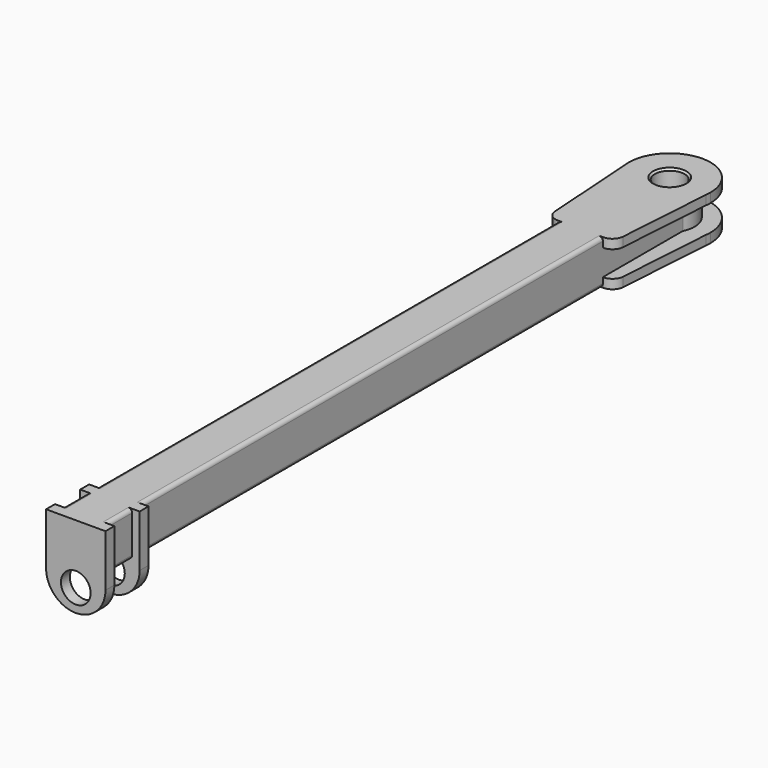
from build123d import *

# Parameters (mm, degrees)
F0_W      = 120
F0_H      = 120
F0_W_2    = 100
F0_H_2    = 100
F1_DEPTH  = 1000
F2_R      = 67.5
F3_DEPTH  = 120
F4_R      = 40
F5_DEPTH  = 120
F7_DEPTH  = 25
F9_DEPTH  = 25
F10_R     = 40
F11_DEPTH = 160
F12_W     = 30
F12_H     = 220
F13_DEPTH = 140
F14_W     = 30
F14_H     = 220
F15_DEPTH = 20
F16_W     = 30
F16_H     = 220
F17_DEPTH = 140
F18_W     = 30
F18_H     = 220
F19_DEPTH = 20
F20_R     = 40
F21_DEPTH = 145
F22_R     = 10
F23_R     = 79.99999
F24_R     = 30
F25_SIZE  = 5


# Not quite as in the source:
# - a fillet or chamfer is up to 0.001 mm smaller than in the source, because OpenCascade refuses the exact size


with BuildPart() as f1:
    # F0 (on Front) → F1 (new body, symmetric)
    with BuildSketch(Plane.XZ):
        Rectangle(F0_W, F0_H)
        Rectangle(F0_W_2, F0_H_2, mode=Mode.SUBTRACT)
    extrude(amount=F1_DEPTH, both=True)

    # F2 (on face) → F3 (join)
    with BuildSketch(Plane.XY.offset(60)):
        with Locations((0, 1000)):
            Circle(F2_R)
    extrude(amount=-F3_DEPTH)

    # F4 (on face) → F5 (cut)
    with BuildSketch(Plane.XY.offset(60)):
        with Locations((0, 1000)):
            Circle(F4_R)
    extrude(amount=-F5_DEPTH, mode=Mode.SUBTRACT)

    # F6 (on face) → F7 (join)
    with BuildSketch(Plane.XY.offset(60)):
        with BuildLine():
            Line((109.0265486726, 985.3982300885), (110, 1000))
            ThreePointArc((110, 1000), (0, 1110), (-110, 1000))
            Line((-110, 1000), (-109.0265486726, 985.3982300885))
            ThreePointArc((-109.0265486726, 985.3982300885), (0, 890), (109.0265486726, 985.3982300885))
        make_face()
        with BuildLine():
            ThreePointArc((109.0265486726, 985.3982300885), (109.7563673642, 992.6829088424), (110, 1000))
            Line((110, 1000), (109.0265486726, 985.3982300885))
        make_face()
        with BuildLine():
            Line((-109.0265486726, 985.3982300885), (-110, 1000))
            ThreePointArc((-110, 1000), (-109.7563673642, 992.6829088424), (-109.0265486726, 985.3982300885))
        make_face()
        with BuildLine():
            Line((90, 700), (109.0265486726, 985.3982300885))
            ThreePointArc((109.0265486726, 985.3982300885), (0, 890), (-109.0265486726, 985.3982300885))
            Line((-109.0265486726, 985.3982300885), (-90, 700))
            Line((-90, 700), (90, 700))
        make_face()
    extrude(amount=-F7_DEPTH)

    # F8 (on face) → F9 (join)
    with BuildSketch(Plane(origin=(0, 0, -60), x_dir=(1, 0, 0), z_dir=(0, 0, -1))):
        with BuildLine():
            Line((109.0265486726, -985.3982300885), (110, -1000))
            ThreePointArc((110, -1000), (109.7563673642, -992.6829088424), (109.0265486726, -985.3982300885))
        make_face()
        with BuildLine():
            ThreePointArc((-109.7502513746, -992.5917395282), (-3.706234531, -1109.9375451136), (110, -1000))
            Line((110, -1000), (109.0265486726, -985.3982300885))
            ThreePointArc((109.0265486726, -985.3982300885), (-3.6149109138, -890.0594141407), (-109.7502513746, -992.5917395282))
        make_face()
        with BuildLine():
            ThreePointArc((-109.7502513746, -992.5917395282), (-3.6149109138, -890.0594141407), (109.0265486726, -985.3982300885))
            Line((109.0265486726, -985.3982300885), (90, -700))
            Line((90, -700), (-90, -700))
            Line((-90, -700), (-109.7502513746, -992.5917395282))
        make_face()
    extrude(amount=-F9_DEPTH)

    # F10 (on face) → F11 (cut)
    with BuildSketch(Plane(origin=(0, 0, -60), x_dir=(1, 0, 0), z_dir=(0, 0, -1))):
        with Locations((0, -1000)):
            Circle(F10_R)
    extrude(amount=-F11_DEPTH, mode=Mode.SUBTRACT)

    # F12 (on face) → F13 (join)
    with BuildSketch(Plane.YZ.offset(60)):
        with Locations((-870, -50)):
            Rectangle(F12_W, F12_H)
    extrude(amount=-F13_DEPTH)

    # F14 (on face) → F15 (join)
    with BuildSketch(Plane.YZ.offset(60)):
        with Locations((-870, -50)):
            Rectangle(F14_W, F14_H)
    extrude(amount=F15_DEPTH)

    # F16 (on face) → F17 (join)
    with BuildSketch(Plane.YZ.offset(60)):
        with Locations((-985, -50)):
            Rectangle(F16_W, F16_H)
    extrude(amount=-F17_DEPTH)

    # F18 (on face) → F19 (join)
    with BuildSketch(Plane.YZ.offset(60)):
        with Locations((-985, -50)):
            Rectangle(F18_W, F18_H)
    extrude(amount=F19_DEPTH)

    # F20 (on face) → F21 (cut)
    with BuildSketch(Plane.XZ.offset(1000)):
        with Locations((0, -100)):
            Circle(F20_R)
    extrude(amount=-F21_DEPTH, mode=Mode.SUBTRACT)

    # F22
    f22_edges = [f1.edges().sort_by_distance(p)[0] for p in [
        (60, -77.5, 60),
        (60, -77.5, -60),
        (60, -927.5, -60),
        (60, -927.5, 60),
        (-60, -77.5, 60),
        (-60, -927.5, 60),
        (-60, -927.5, -60),
        (-60, -77.5, -60),
    ]]
    fillet(f22_edges, radius=F22_R)

    # F23 (radius 80 in the source; OpenCascade refuses exactly that, so slightly less here)
    f23_edges = [f1.edges().sort_by_distance(p)[0] for p in [
        (-80, -985, -160),
        (80, -985, -160),
        (80, -870, -160),
        (-80, -870, -160),
    ]]
    fillet(f23_edges, radius=F23_R)

    # F24
    f24_edges = [f1.edges().sort_by_distance(p)[0] for p in [
        (-90, 700, -47.5),
        (-90, 700, 47.5),
        (90, 700, -47.5),
        (90, 700, 47.5),
    ]]
    fillet(f24_edges, radius=F24_R)

    # F25
    f25_edges = [f1.edges().sort_by_distance(p)[0] for p in [
        (-40, 1000, 60),
        (-40, 1000, -60),
    ]]
    chamfer(f25_edges, length=F25_SIZE)


solid = f1.part
